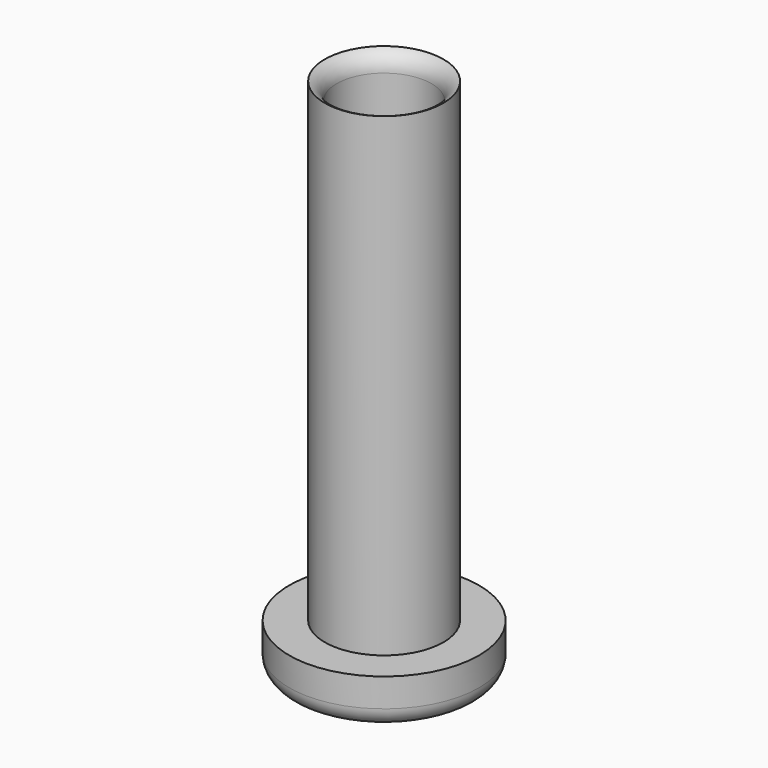
from build123d import *

# Parameters (mm, degrees)
F0_R     = 10
F0_R_2   = 6.25
F1_DEPTH = 5
F0_R_3   = 5
F2_DEPTH = 55
F3_DEPTH = 51


# Not quite as in the source:
# - a fillet or chamfer that OpenCascade refuses, or shapes differently, is made with other operations: its cross-section is extruded or revolved along the edge and cut away or added


with BuildPart() as f1:
    # F0 (on Top) → F1 (new body)
    with BuildSketch(Plane.XY):
        Circle(F0_R)
        Circle(F0_R_2, mode=Mode.SUBTRACT)
    extrude(amount=F1_DEPTH)

    # F0 (on Top) → F2 (join)
    with BuildSketch(Plane.XY):
        Circle(F0_R_2)
        Circle(F0_R_3, mode=Mode.SUBTRACT)
    extrude(amount=F2_DEPTH)

    # F0 (on Top) → F3 (cut)
    with BuildSketch(Plane.XY):
        Circle(F0_R_3)
    extrude(amount=F3_DEPTH, mode=Mode.SUBTRACT)

    # F4: fillet of radius 2 on 3 edges, made by hand

    # F4_s1 → F4_t2 (revolve, cut)
    with BuildSketch(Plane.XZ):
        with BuildLine():
            ThreePointArc((5, 2), (5.5857864376, 0.5857864376), (7, 0))
            Line((7, 0), (5, 0))
            Line((5, 0), (5, 2))
        make_face()
    revolve(axis=Axis((0, 0, 0), (0, 0, 1)), mode=Mode.SUBTRACT)

    # F4_s3 → F4_t4 (revolve, cut)
    with BuildSketch(Plane.XZ):
        with BuildLine():
            ThreePointArc((6.25, 55), (5.3416876048, 54.263984367), (5, 53.1459503782))
            Line((5, 53.1459503782), (5, 55))
            Line((5, 55), (6.25, 55))
        make_face()
    revolve(axis=Axis((0, 0, 55), (0, 0, 1)), mode=Mode.SUBTRACT)

    # F4_s5 → F4_t6 (revolve, cut)
    with BuildSketch(Plane.XZ):
        with BuildLine():
            ThreePointArc((10, 2), (9.4142135624, 0.5857864376), (8, 0))
            Line((8, 0), (10, 0))
            Line((10, 0), (10, 2))
        make_face()
    revolve(axis=Axis((0, 0, 0), (0, 0, 1)), mode=Mode.SUBTRACT)


solid = f1.part
